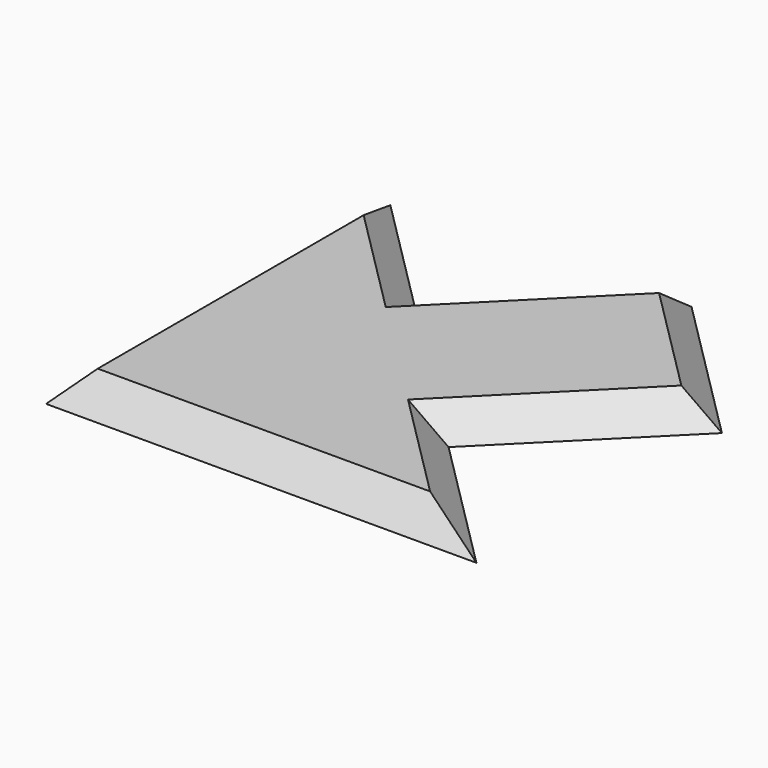
from build123d import *

# Parameters (mm, degrees)
F1_DEPTH = 2
F2_SIZE  = 1.99999


# Not quite as in the source:
# - a fillet or chamfer is up to 0.001 mm smaller than in the source, because OpenCascade refuses the exact size


with BuildPart() as f1:
    # F0 (on Top) → F1 (new body)
    with BuildSketch(Plane.XY):
        Polygon((0, 30), (0, 0), (30, 0), (20.2933432917, 9.7066567083), (30.880029875, 20.2933432917), (20.2933432917, 30.880029875), (9.7066567083, 20.2933432917), align=None)
    extrude(amount=F1_DEPTH)

    # F2 (size 2 in the source; OpenCascade refuses exactly that, so slightly less here)
    f2_edges = [f1.edges().sort_by_distance(p)[0] for p in [
        (25.586687, 15, 2),
        (15, 25.586687, 2),
        (25.146672, 4.853328, 2),
        (15, 0, 2),
        (0, 15, 2),
        (4.853328, 25.146672, 2),
        (25.586687, 25.586687, 2),
    ]]
    chamfer(f2_edges, length=F2_SIZE)


solid = f1.part
